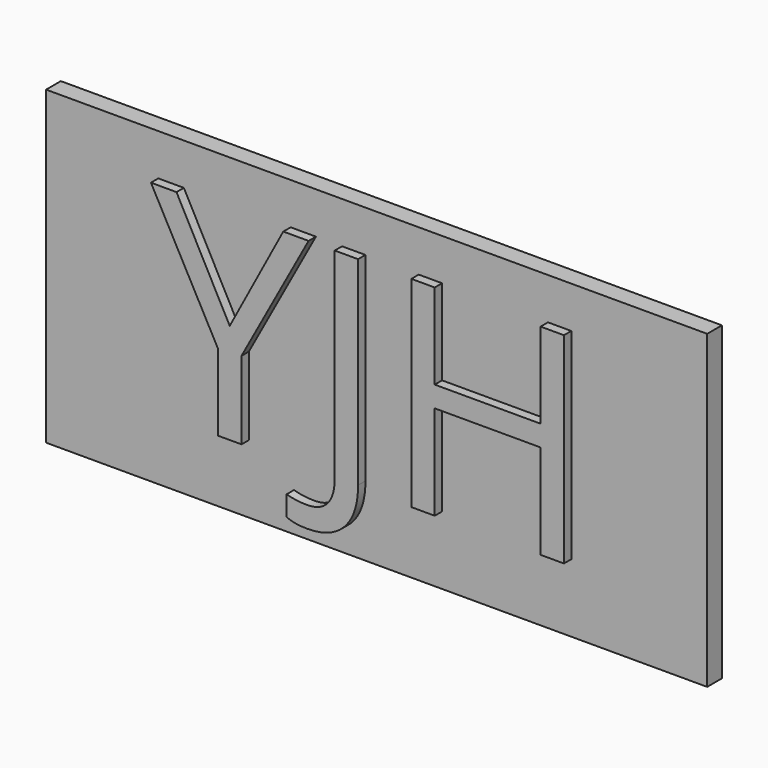
from build123d import *

# Parameters (mm, degrees)
F0_W         = 91.1634713411
F0_H         = 42.8625009954
F1_DEPTH     = 2.54
F2_TEXT_SIZE = 38.8151966035
F3_DEPTH     = 1.27


# Not quite as in the source:
# - Text() gives the source's letters only with a copy of the font that has no kerning and outlines rounded to 1/6400 em; it was checked with that copy


with BuildPart() as f1:
    # F0 (on Front) → F1 (new body)
    with BuildSketch(Plane.XZ):
        with Locations((45.5817356706, 21.4312504977)):
            Rectangle(F0_W, F0_H)
    extrude(amount=F1_DEPTH)

    # F2 (on face) → F3 (join)
    with BuildSketch(Plane.XZ.offset(2.54)):
        with Locations((15.476278495, 9.4053824432)):
            Text('YJH', F2_TEXT_SIZE, font='Open Sans', text_align=(TextAlign.LEFT, TextAlign.BOTTOM))
    extrude(amount=F3_DEPTH)


solid = f1.part
